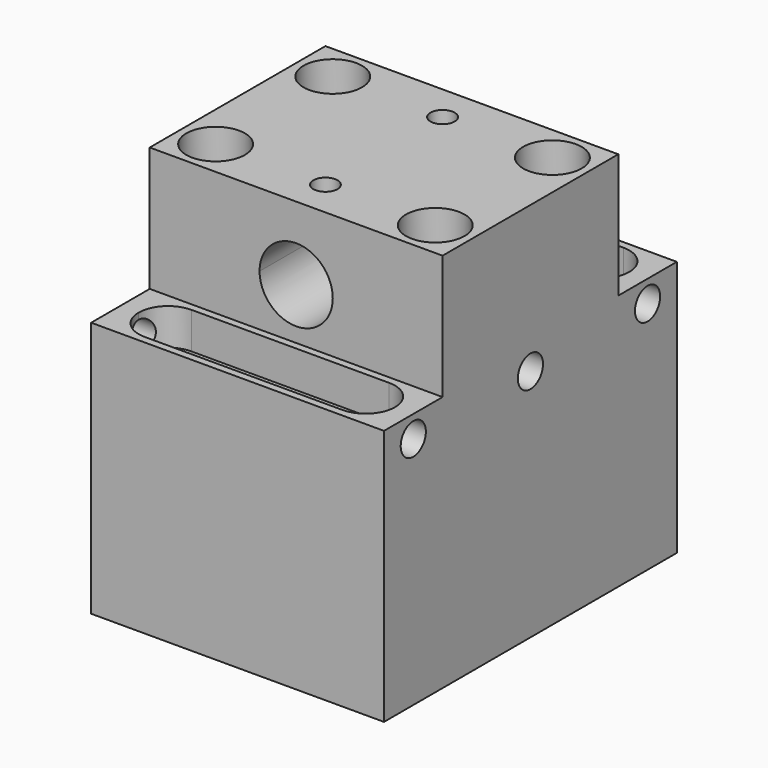
from build123d import *
from build123d import SkipClean  # not in build123d's __all__

# Parameters (mm, degrees)
F0_W      = 40
F0_H      = 30
F1_DEPTH  = 52
F2_R      = 5
F3_DEPTH  = 20
F4_R      = 1.65
F5_DEPTH  = 10
F6_R      = 2.5
F7_DEPTH  = 52.001
F8_R      = 4
F9_DEPTH  = 5
F10_W     = 40
F10_H     = 35
F11_DEPTH = 10
F12_W     = 40
F12_H     = 35
F13_DEPTH = 10
F15_DEPTH = 5
F16_R     = 2.15
F17_DEPTH = 40.001
F18_R     = 5
F19_DEPTH = 40.001
F20_R     = 6
F21_DEPTH = 1
F22_R     = 2.25
F23_DEPTH = 15.5358573251


with BuildPart() as f1:
    # F0 (on Top) → F1 (new body)
    with BuildSketch(Plane.XY):
        with Locations((20, 15)):
            Rectangle(F0_W, F0_H)
    extrude(amount=F1_DEPTH)

    # F2 (on face) → F3 (cut)
    with BuildSketch(Plane.XZ):
        with Locations((20, 42)):
            Circle(F2_R)
    extrude(amount=-F3_DEPTH, mode=Mode.SUBTRACT)

    # F4 (on face) → F5 (cut)
    with BuildSketch(Plane.XY.offset(52)):
        with Locations((20, 5)):
            Circle(F4_R)
        with Locations((20, 25)):
            Circle(F4_R)
    extrude(amount=-F5_DEPTH, mode=Mode.SUBTRACT)

    # F6 (on face) → F7 (cut, through all)
    with BuildSketch(Plane.XY.offset(52)):
        with Locations((5, 5)):
            Circle(F6_R)
        with Locations((5, 25)):
            Circle(F6_R)
        with Locations((35, 5)):
            Circle(F6_R)
        with Locations((35, 25)):
            Circle(F6_R)
    extrude(amount=-F7_DEPTH, mode=Mode.SUBTRACT)

    # F8 (on face) → F9 (cut)
    with BuildSketch(Plane.XY.offset(52)):
        with Locations((5, 25)):
            Circle(F8_R)
        with Locations((5, 5)):
            Circle(F8_R)
        with Locations((35, 25)):
            Circle(F8_R)
        with Locations((35, 5)):
            Circle(F8_R)
    extrude(amount=-F9_DEPTH, mode=Mode.SUBTRACT)

    # F10 (on face) → F11 (join)
    with BuildSketch(Plane.XZ):
        with Locations((20, 17.5)):
            Rectangle(F10_W, F10_H)
    extrude(amount=F11_DEPTH)

    # F12 (on face) → F13 (join)
    with BuildSketch(Plane(origin=(0, 30, 0), x_dir=(-1, 0, 0), z_dir=(0, 1, 0))):
        with Locations((-20, 17.5)):
            Rectangle(F12_W, F12_H)
    extrude(amount=F13_DEPTH)

    # F14 (on face) → F15 (cut)
    with BuildSketch(Plane.XY.offset(35)):
        with BuildLine():
            Line((6.5, 31), (33.5, 31))
            ThreePointArc((33.5, 31), (36.3284271247, 32.1715728753), (37.5, 35))
            ThreePointArc((37.5, 35), (36.3284271247, 37.8284271247), (33.5, 39))
            Line((33.5, 39), (6.5, 39))
            ThreePointArc((6.5, 39), (3.6715728753, 37.8284271247), (2.5, 35))
            ThreePointArc((2.5, 35), (3.6715728753, 32.1715728753), (6.5, 31))
        make_face()
        with BuildLine():
            Line((6.5, -9), (33.5, -9))
            ThreePointArc((33.5, -9), (36.3284271247, -7.8284271247), (37.5, -5))
            ThreePointArc((37.5, -5), (36.3284271247, -2.1715728753), (33.5, -1))
            Line((33.5, -1), (6.5, -1))
            ThreePointArc((6.5, -1), (3.6715728753, -2.1715728753), (2.5, -5))
            ThreePointArc((2.5, -5), (3.6715728753, -7.8284271247), (6.5, -9))
        make_face()
    extrude(amount=-F15_DEPTH, mode=Mode.SUBTRACT)

    # F16 (on face) → F17 (cut, through all)
    with BuildSketch(Plane(origin=(0, 0, 0), x_dir=(0, -1, 0), z_dir=(-1, 0, 0))):
        with Locations((-15, 32)):
            Circle(F16_R)
        with Locations((-35, 32)):
            Circle(F16_R)
        with Locations((5, 32)):
            Circle(F16_R)
    extrude(amount=-F17_DEPTH, mode=Mode.SUBTRACT)

    # F18 (on face) → F19 (cut, through all)
    with BuildSketch(Plane(origin=(0, 30, 0), x_dir=(-1, 0, 0), z_dir=(0, 1, 0))):
        with Locations((-20, 42)):
            Circle(F18_R)
    with SkipClean():  # cleaning this boolean's faces spoils the solid; the shape is the same uncleaned
        extrude(amount=-F19_DEPTH, mode=Mode.SUBTRACT)

    # F20 (on face) → F21 (cut)
    with BuildSketch(Plane(origin=(0, 30, 0), x_dir=(-1, 0, 0), z_dir=(0, 1, 0))):
        with Locations((-20, 42)):
            Circle(F20_R)
    with SkipClean():  # cleaning this boolean's faces spoils the solid; the shape is the same uncleaned
        extrude(amount=-F21_DEPTH, mode=Mode.SUBTRACT)

    # F22 (on face) → F23 (cut, through all)
    with BuildSketch(Plane(origin=(0, 0, 0), x_dir=(0, -1, 0), z_dir=(-1, 0, 0))):
        with Locations((-15, 42)):
            Circle(F22_R)
    with SkipClean():  # cleaning this boolean's faces spoils the solid; the shape is the same uncleaned
        extrude(amount=-F23_DEPTH, mode=Mode.SUBTRACT)


solid = f1.part
